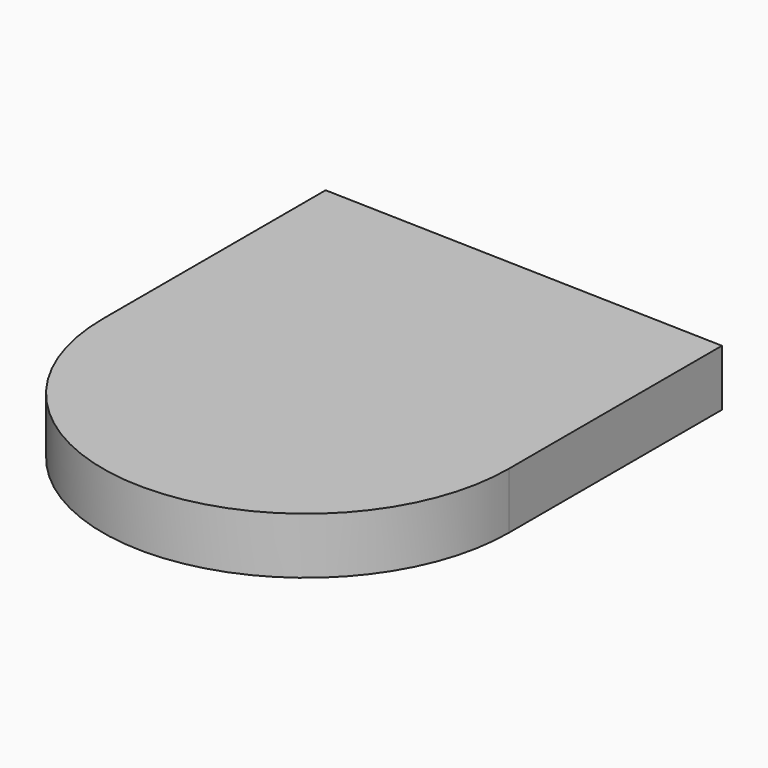
from build123d import *

# Parameters (mm, degrees)
F1_DEPTH       = 12.7
F2_TEXT_SIZE   = 10.0864770098
F2_TEXT_SIZE_2 = 9.5016620536
F3_DEPTH       = 5.08


# Not quite as in the source:
# - Text() gives the source's letters only with a copy of the font that has no kerning and outlines rounded to 1/6400 em; it was checked with that copy


with BuildPart() as f1:
    # F0 (on Top) → F1 (new body)
    with BuildSketch(Plane.XY):
        with BuildLine():
            Line((-124.4647428393, 34.3671515584), (-124.4647428393, -28.3059184439))
            ThreePointArc((-124.4647428393, -28.3059184439), (-78.7660829354, -74.0045783479), (-33.0674230315, -28.3059184439))
            Line((-33.0674230315, -28.3059184439), (-33.0674230315, 31.6586345434))
            Line((-33.0674230315, 31.6586345434), (-124.4647428393, 34.3671515584))
        make_face()
    extrude(amount=F1_DEPTH)

    # F2 (on face) → F3 (join)
    with BuildSketch(Plane(origin=(0, 0, 0), x_dir=(1, 0, 0), z_dir=(0, 0, -1))):
        with Locations((-110.544487834, 42.4736589193)):
            Text('Helen Garcia', F2_TEXT_SIZE, font='Open Sans', text_align=(TextAlign.LEFT, TextAlign.BOTTOM))
        with Locations((-102.7921885252, -21.6654259712)):
            Text('1987-2016', F2_TEXT_SIZE_2, font='Open Sans', text_align=(TextAlign.LEFT, TextAlign.BOTTOM))
    extrude(amount=F3_DEPTH)


solid = f1.part
